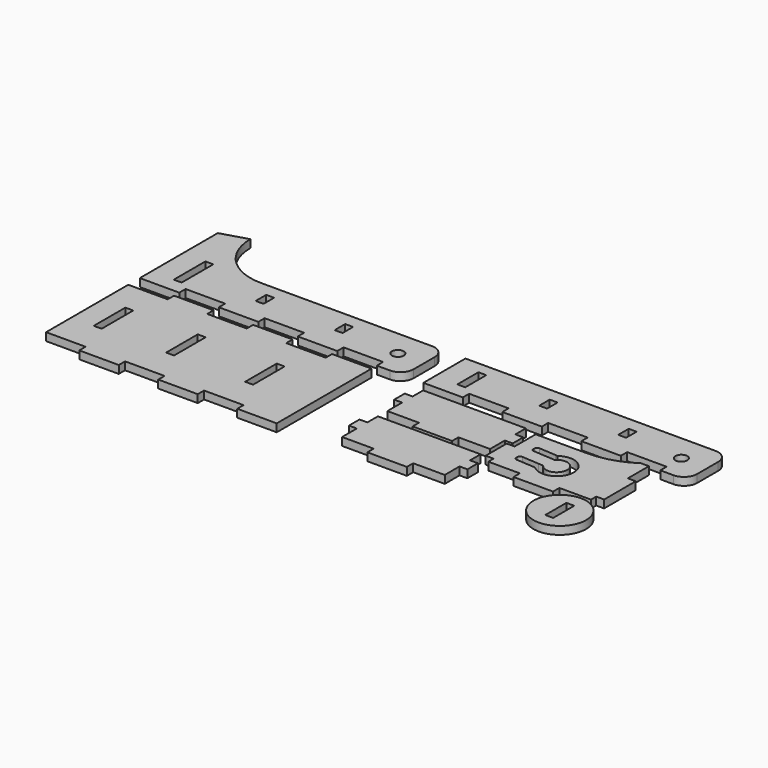
from build123d import *

# Parameters (mm, degrees)
F1_R     = 10
F1_W     = 3
F1_H     = 10
F2_DEPTH = 3
F1_H_2   = 5
F1_R_2   = 2.25
F1_H_3   = 15


# Not quite as in the source:
# - a feature names something its author has since deleted; it is built from what else it names


with BuildPart() as f2:
    # F1 (on Top) → F2 (new body)
    with BuildSketch(Plane.XY):
        with Locations((190.4685690403, -38.7000021338)):
            Circle(F1_R)
        with Locations((190.4685690403, -38.7000021338)):
            Rectangle(F1_W, F1_H, mode=Mode.SUBTRACT)
    extrude(amount=F2_DEPTH)


with BuildPart() as f2b:
    # F1 (on Top) → F2, piece 2 (new body)
    with BuildSketch(Plane.XY):
        with BuildLine():
            Line((154.3685435057, -25.0202883035), (154.3685435057, -27.5202883035))
            Line((154.3685435057, -27.5202883035), (166.3685435057, -27.5202883035))
            Line((166.3685435057, -27.5202883035), (166.3685435057, -30.5202883035))
            Line((166.3685435057, -30.5202883035), (173.8685435057, -30.5202883035))
            Line((173.8685435057, -30.5202883035), (181.3685435057, -30.5202883035))
            Line((181.3685435057, -30.5202883035), (181.3685435057, -27.5202883035))
            Line((181.3685435057, -27.5202883035), (193.3685435057, -27.5202883035))
            Line((193.3685435057, -27.5202883035), (193.3685435057, -25.0202883035))
            Line((193.3685435057, -25.0202883035), (196.3685435057, -25.0202883035))
            Line((196.3685435057, -25.0202883035), (196.3685435057, -10.0202883035))
            Line((196.3685435057, -10.0202883035), (193.3685435057, -10.0202883035))
            Line((193.3685435057, -10.0202883035), (193.3685435057, -0.0202883035))
            Line((193.3685435057, -0.0202883035), (190.3685435057, -0.0202883035))
            ThreePointArc((190.3685435057, -0.0202883035), (182.4890133305, -3.7428387253), (173.8685435057, -5.0202883035))
            Line((173.8685435057, -5.0202883035), (154.3685435057, -5.0202883035))
            Line((154.3685435057, -5.0202883035), (154.3685435057, -15.0202883035))
            Line((154.3685435057, -15.0202883035), (151.3685435057, -15.0202883035))
            Line((151.3685435057, -15.0202883035), (151.3685435057, -25.0202883035))
            Line((151.3685435057, -25.0202883035), (154.3685435057, -25.0202883035))
        make_face()
        with BuildLine():
            Line((169.0201585277, -14.3506918411), (167.1467590467, -14.2266580037))
            Line((167.1467590467, -14.2266580037), (160.6609587085, -13.7972468117))
            ThreePointArc((160.6609587085, -13.7972468117), (159.9747461278, -13.4582796573), (159.7292065321, -12.7333681147))
            Line((159.7292065321, -12.7333681147), (159.7622381623, -12.2344603964))
            ThreePointArc((159.7622381623, -12.2344603964), (160.1012053166, -11.5482478157), (160.8261168592, -11.30270822))
            Line((160.8261168592, -11.30270822), (167.3119171975, -11.7321194121))
            Line((167.3119171975, -11.7321194121), (168.1567556224, -11.7880543864))
            ThreePointArc((168.1567556224, -11.7880543864), (178.4564784175, -17.480924089), (167.4961230192, -21.766208753))
            Line((167.4961230192, -21.766208753), (166.6512845944, -21.7102737787))
            Line((166.6512845944, -21.7102737787), (160.1654842561, -21.2808625866))
            ThreePointArc((160.1654842561, -21.2808625866), (159.4792716754, -20.9418954323), (159.2337320797, -20.2169838897))
            Line((159.2337320797, -20.2169838897), (159.2667637099, -19.7180761713))
            ThreePointArc((159.2667637099, -19.7180761713), (159.6057308643, -19.0318635907), (160.3306424069, -18.786323995))
            Line((160.3306424069, -18.786323995), (166.8164427452, -19.215735187))
            Line((166.8164427452, -19.215735187), (168.6898422261, -19.3397690244))
            ThreePointArc((168.6898422261, -19.3397690244), (175.9619398259, -17.3157659382), (169.0201585277, -14.3506918411))
        make_face(mode=Mode.SUBTRACT)
    extrude(amount=F2_DEPTH)


with BuildPart() as f2c:
    # F1 (on Top) → F2, piece 3 (new body)
    with BuildSketch(Plane.XY):
        with BuildLine():
            Line((107.6887845993, 20), (107.6887845993, 0))
            Line((107.6887845993, 0), (122.6887845993, 0))
            Line((122.6887845993, 0), (122.6887845993, 3))
            Line((122.6887845993, 3), (137.6887845993, 3))
            Line((137.6887845993, 3), (137.6887845993, 0))
            Line((137.6887845993, 0), (152.6887845993, 0))
            Line((152.6887845993, 0), (152.6887845993, 3))
            Line((152.6887845993, 3), (167.6887845993, 3))
            Line((167.6887845993, 3), (167.6887845993, 0))
            Line((167.6887845993, 0), (182.6887845993, 0))
            Line((182.6887845993, 0), (182.6887845993, 3))
            Line((182.6887845993, 3), (197.6887845993, 3))
            Line((197.6887845993, 3), (197.6887845993, 0))
            Line((197.6887845993, 0), (202.6887845993, 0))
            ThreePointArc((202.6887845993, 0), (206.2243185052, 1.4644660941), (207.6887845993, 5))
            Line((207.6887845993, 5), (207.6887845993, 15))
            ThreePointArc((207.6887845993, 15), (206.2243185052, 18.5355339059), (202.6887845993, 20))
            Line((202.6887845993, 20), (137.6887845993, 20))
            Line((137.6887845993, 20), (107.6887845993, 20))
        make_face()
        with Locations((117.6887845993, 10.5)):
            Rectangle(F1_W, F1_H, mode=Mode.SUBTRACT)
        with Locations((145.1887845993, 12.5)):
            Rectangle(F1_W, F1_H_2, mode=Mode.SUBTRACT)
        with Locations((175.1887845993, 12.5)):
            Rectangle(F1_W, F1_H_2, mode=Mode.SUBTRACT)
        with Locations((197.6887845993, 10)):
            Circle(F1_R_2, mode=Mode.SUBTRACT)
    extrude(amount=F2_DEPTH)


with BuildPart() as f2d:
    # F1 (on Top) → F2, piece 4 (new body)
    with BuildSketch(Plane.XY):
        Polygon((15, -5.493568331), (0, -5.493568331), (0, -24.993568331), (0, -44.493568331), (15, -44.493568331), (15, -47.493568331), (30, -47.493568331), (30, -44.493568331), (45, -44.493568331), (45, -47.493568331), (60, -47.493568331), (60, -44.493568331), (75, -44.493568331), (75, -47.493568331), (90, -47.493568331), (90, -44.493568331), (90, -24.993568331), (90, -5.493568331), (90, -2.493568331), (75, -2.493568331), (75, -5.493568331), (60, -5.493568331), (60, -2.493568331), (45, -2.493568331), (45, -5.493568331), (30, -5.493568331), (30, -2.493568331), (15, -2.493568331), align=None)
        with Locations((10, -24.993568331)):
            Rectangle(F1_W, F1_H_3, mode=Mode.SUBTRACT)
        with Locations((37.5, -24.993568331)):
            Rectangle(F1_W, F1_H_3, mode=Mode.SUBTRACT)
        with Locations((67.5, -24.993568331)):
            Rectangle(F1_W, F1_H_3, mode=Mode.SUBTRACT)
    extrude(amount=F2_DEPTH)


with BuildPart() as f2e:
    # F1 (on Top) → F2, piece 5 (new body)
    with BuildSketch(Plane.XY):
        Polygon((130.1870310709, -3.8339694942), (110.6870310709, -3.8339694942), (110.6870310709, -8.8339694942), (107.6870310709, -8.8339694942), (107.6870310709, -13.8339694942), (110.6870310709, -13.8339694942), (110.6870310709, -20.8339694942), (122.6870310709, -20.8339694942), (122.6870310709, -23.8339694942), (130.1870310709, -23.8339694942), (137.6870310709, -23.8339694942), (137.6870310709, -20.8339694942), (149.6870310709, -20.8339694942), (149.6870310709, -13.8339694942), (152.6870310709, -13.8339694942), (152.6870310709, -8.8339694942), (149.6870310709, -8.8339694942), (149.6870310709, -3.8339694942), align=None)
    extrude(amount=F2_DEPTH)


with BuildPart() as f2f:
    # F1 (on Top) → F2, piece 6 (new body)
    with BuildSketch(Plane.XY):
        Polygon((130.1044501066, -25.2247648239), (110.6044501066, -25.2247648239), (110.6044501066, -30.2247648239), (107.6044501066, -30.2247648239), (107.6044501066, -35.2247648239), (110.6044501066, -35.2247648239), (110.6044501066, -42.2247648239), (122.6044501066, -42.2247648239), (122.6044501066, -45.2247648239), (130.1044501066, -45.2247648239), (137.6044501066, -45.2247648239), (137.6044501066, -42.2247648239), (149.6044501066, -42.2247648239), (149.6044501066, -35.2247648239), (152.6044501066, -35.2247648239), (152.6044501066, -30.2247648239), (149.6044501066, -30.2247648239), (149.6044501066, -25.2247648239), align=None)
    extrude(amount=F2_DEPTH)


with BuildPart() as f2g:
    # F1 (on Top) → F2, piece 7 (new body)
    with BuildSketch(Plane.XY):
        with BuildLine():
            ThreePointArc((30, 20), (15.8578643763, 25.8578643763), (10, 40))
            Line((10, 40), (0, 37))
            Line((0, 37), (0, 0))
            Line((0, 0), (15, 0))
            Line((15, 0), (15, 3))
            Line((15, 3), (30, 3))
            Line((30, 3), (30, 0))
            Line((30, 0), (45, 0))
            Line((45, 0), (45, 3))
            Line((45, 3), (60, 3))
            Line((60, 3), (60, 0))
            Line((60, 0), (75, 0))
            Line((75, 0), (75, 3))
            Line((75, 3), (90, 3))
            Line((90, 3), (90, 0))
            Line((90, 0), (95, 0))
            ThreePointArc((95, 0), (98.5355339059, 1.4644660941), (100, 5))
            Line((100, 5), (100, 15))
            ThreePointArc((100, 15), (98.5355339059, 18.5355339059), (95, 20))
            Line((95, 20), (30, 20))
        make_face()
        with Locations((10, 13)):
            Rectangle(F1_W, F1_H_3, mode=Mode.SUBTRACT)
        with Locations((37.5, 12.5)):
            Rectangle(F1_W, F1_H_2, mode=Mode.SUBTRACT)
        with Locations((67.5, 12.5)):
            Rectangle(F1_W, F1_H_2, mode=Mode.SUBTRACT)
        with Locations((90, 10)):
            Circle(F1_R_2, mode=Mode.SUBTRACT)
    extrude(amount=F2_DEPTH)


solid = Compound([f2.part, f2b.part, f2c.part, f2d.part, f2e.part, f2f.part, f2g.part])
